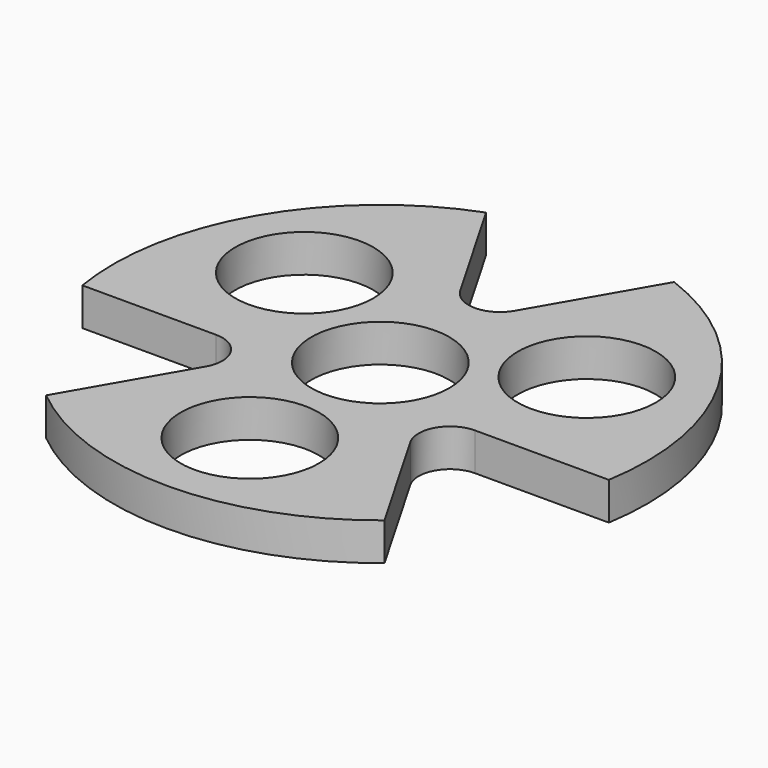
from build123d import *

# Parameters (mm, degrees)
F0_R            = 42.5
F0_R_2          = 11
F1_DEPTH        = 6
F3_DEPTH        = 25
F3_COPIES_COUNT = 3
F4_R            = 5


# Not quite as in the source:
# - a pattern or mirror of a feature is missing from the dataset's text; its kind, count and spacing are read off the source's solid


with BuildPart() as f1:
    # F0 (on Top) → F1 (new body)
    with BuildSketch(Plane.XY):
        Circle(F0_R)
        with Locations((0, -25.9807621135)):
            Circle(F0_R_2, mode=Mode.SUBTRACT)
        with Locations((-22.5, 12.9903810568)):
            Circle(F0_R_2, mode=Mode.SUBTRACT)
        Circle(F0_R_2, mode=Mode.SUBTRACT)
        with Locations((22.5, 12.9903810568)):
            Circle(F0_R_2, mode=Mode.SUBTRACT)
    extrude(amount=F1_DEPTH)

    # F2 (on face) → F3 (cut)
    with BuildSketch(Plane.XY.offset(6)):
        with BuildLine():
            Line((11.9734825652, -6.9128933822), (26.9537505179, -32.8594785872))
            ThreePointArc((26.9537505179, -32.8594785872), (36.8060796608, -21.25), (41.9340184705, -6.9128933822))
            Line((41.9340184705, -6.9128933822), (11.9734825652, -6.9128933822))
        make_face()
    f3 = extrude(amount=-F3_DEPTH, mode=Mode.SUBTRACT)

    # F3_copies: F3 ×3 about axis
    f3_copies_axis = Axis((0, 0, 0), (0, 0, 1))
    for i in range(1, F3_COPIES_COUNT):
        add(f3.rotate(f3_copies_axis, i * 360 / F3_COPIES_COUNT), mode=Mode.SUBTRACT)

    # F4
    f4_edges = [f1.edges().sort_by_distance(p)[0] for p in [
        (11.973483, -6.912893, 3),
        (0, 13.825787, 3),
        (-11.973483, -6.912893, 3),
    ]]
    fillet(f4_edges, radius=F4_R)


solid = f1.part
